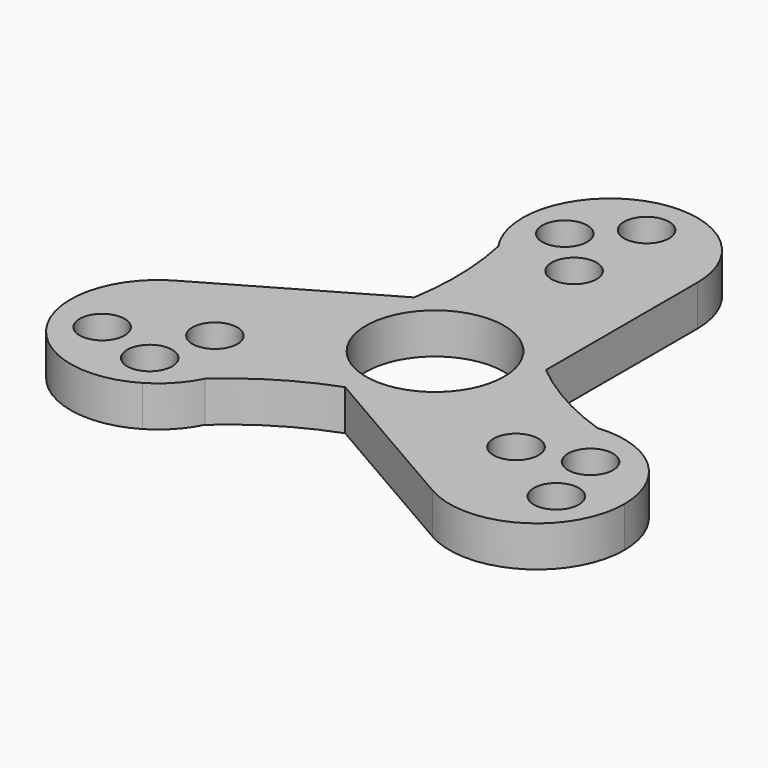
from build123d import *

# Parameters (mm, degrees)
F0_R     = 3.6
F0_R_2   = 11.05
F1_DEPTH = 6.5


# Not quite as in the source:
# - a feature names something its author has since deleted; it is built from what else it names


with BuildPart() as f1:
    # F0 (on Top) → F1 (new body)
    with BuildSketch(Plane.XY):
        with BuildLine():
            ThreePointArc((-23.0209464524, -29.3076083822), (-19.9383676627, -26.8167802289), (-17.6773098575, -23.5619170235))
            ThreePointArc((-17.6773098575, -23.5619170235), (-20.4709038775, -26.3215082368), (-23.0209464524, -29.3076083822))
        make_face()
        with BuildLine():
            ThreePointArc((-2.5600533635, -14.3957456382), (-1.63787321, -14.0667717582), (-0.7089513801, -13.7573460272))
            ThreePointArc((-0.7089513801, -13.7573460272), (-3.7381834506, -13.2395644299), (-6.5814605839, -12.0733226612))
            Line((-6.5814605839, -12.0733226612), (-2.5600533635, -14.3957456382))
        make_face()
        with BuildLine():
            ThreePointArc((-0.7089513801, -13.7573460272), (3.2568779095, -13.4262355322), (6.9693155956, -11.9926238203))
            ThreePointArc((6.9693155956, -11.9926238203), (3.0926272048, -12.7115843783), (-0.7089513801, -13.7573460272))
        make_face()
        with BuildLine():
            ThreePointArc((29.002813969, -3.3554863963), (22.1605329653, -5.9872334975), (17.5863384821, -11.7160769207))
            ThreePointArc((17.5863384821, -11.7160769207), (17.1389450218, -21.6742013703), (23.4307313902, -29.4058136055))
            ThreePointArc((23.4307313902, -29.4058136055), (37.4314802249, -29.4071108103), (44.4322291397, -17.282322802))
            ThreePointArc((44.4322291397, -17.282322802), (39.8127458528, -6.8897337985), (29.002813969, -3.3554863963))
        make_face()
        with Locations((24.2079713773, -13.6886037443)):
            Circle(F0_R, mode=Mode.SUBTRACT)
        with Locations((36.4874702709, -20.9787380615)):
            Circle(F0_R, mode=Mode.SUBTRACT)
        with Locations((33.9983616409, -11.0225966846)):
            Circle(F0_R, mode=Mode.SUBTRACT)
        with BuildLine():
            ThreePointArc((-23.0209464524, -29.3076083822), (-20.4709038775, -26.3215082368), (-17.6773098575, -23.5619170235))
            ThreePointArc((-17.6773098575, -23.5619170235), (-16.5669328393, -20.5090534106), (-16.1900430763, -17.2824658218))
            ThreePointArc((-16.1900430763, -17.2824658218), (-16.8601676515, -13.0029306649), (-18.8063889562, -9.1330843193))
            ThreePointArc((-18.8063889562, -9.1330843193), (-27.0153338433, -3.6471725985), (-36.8032431016, -4.9428716054))
            ThreePointArc((-36.8032431016, -4.9428716054), (-42.3755818337, -24.1754075155), (-23.0209464524, -29.3076083822))
        make_face()
        with Locations((-26.552398323, -23.5003339555)):
            Circle(F0_R, mode=Mode.SUBTRACT)
        with Locations((-36.419223994, -20.6778945734)):
            Circle(F0_R, mode=Mode.SUBTRACT)
        with Locations((-23.9660330315, -13.6886037443)):
            Circle(F0_R, mode=Mode.SUBTRACT)
        with BuildLine():
            ThreePointArc((-11.3063452022, 8.3060793433), (-9.4777201208, 10.4094594589), (-7.2686697166, 12.1089222888))
            Line((-7.2686697166, 12.1089222888), (-11.0034872924, 9.9526243561))
            ThreePointArc((-11.0034872924, 9.9526243561), (-11.1474831305, 9.1279846364), (-11.3063452022, 8.3060793433))
        make_face()
        with BuildLine():
            ThreePointArc((-13.8745275017, -0.137033899), (-12.3890775486, 4.023274448), (-11.3063452022, 8.3060793433))
            ThreePointArc((-11.3063452022, 8.3060793433), (-13.2731105164, 4.292175001), (-13.8745275017, -0.137033899))
        make_face()
        with BuildLine():
            ThreePointArc((6.7990177159, 12.5226532313), (9.6860598983, 9.0919172063), (12.891022892, 5.9561279205))
            ThreePointArc((12.891022892, 5.9561279205), (10.3843499056, 9.7397463301), (6.7990177159, 12.5226532313))
        make_face()
        with BuildLine():
            ThreePointArc((12.891022892, 5.9561279205), (13.810029624, 3.1522495359), (14.1209691729, 0.2180334624))
            Line((14.1209691729, 0.2180334624), (14.1209691729, 4.9018602452))
            ThreePointArc((14.1209691729, 4.9018602452), (13.5013908187, 5.4236214762), (12.891022892, 5.9561279205))
        make_face()
        with BuildLine():
            ThreePointArc((-11.4281301493, 27.3048605939), (-12.4782019744, 31.2955370079), (-13.8789707842, 35.1770310271))
            ThreePointArc((-13.8789707842, 35.1770310271), (-13.2461965273, 31.0564374771), (-11.4281301493, 27.3048605939))
        make_face()
        with BuildLine():
            ThreePointArc((6.7990177159, 12.5226532313), (10.3843499056, 9.7397463301), (12.891022892, 5.9561279205))
            ThreePointArc((12.891022892, 5.9561279205), (13.5013908187, 5.4236214762), (14.1209691729, 4.9018602452))
            Line((14.1209691729, 4.9018602452), (14.1209691729, 35.2180334624))
            ThreePointArc((14.1209691729, 35.2180334624), (4.2629861628, 21.8447879604), (-11.4281301493, 27.3048605939))
            ThreePointArc((-11.4281301493, 27.3048605939), (-10.3964763758, 18.6487931257), (-11.0034872924, 9.9526243561))
            Line((-11.0034872924, 9.9526243561), (-7.2686697166, 12.1089222888))
            ThreePointArc((-7.2686697166, 12.1089222888), (-0.2905931292, 14.2119827431), (6.7990177159, 12.5226532313))
        make_face()
        with BuildLine():
            ThreePointArc((6.9693155956, -11.9926238203), (12.2014668844, -6.8573870227), (14.1209691729, 0.2180334624))
            ThreePointArc((14.1209691729, 0.2180334624), (13.810029624, 3.1522495359), (12.891022892, 5.9561279205))
            ThreePointArc((12.891022892, 5.9561279205), (9.6860598983, 9.0919172063), (6.7990177159, 12.5226532313))
            ThreePointArc((6.7990177159, 12.5226532313), (-0.2905931292, 14.2119827431), (-7.2686697166, 12.1089222888))
            ThreePointArc((-7.2686697166, 12.1089222888), (-9.4777201208, 10.4094594589), (-11.3063452022, 8.3060793433))
            ThreePointArc((-11.3063452022, 8.3060793433), (-12.3890775486, 4.023274448), (-13.8745275017, -0.137033899))
            ThreePointArc((-13.8745275017, -0.137033899), (-11.8255695306, -7.0812961649), (-6.5814605839, -12.0733226612))
            ThreePointArc((-6.5814605839, -12.0733226612), (-3.7381834506, -13.2395644299), (-0.7089513801, -13.7573460272))
            ThreePointArc((-0.7089513801, -13.7573460272), (3.0926272048, -12.7115843783), (6.9693155956, -11.9926238203))
        make_face()
        with Locations((0.1209691729, 0.2180334624)):
            Circle(F0_R_2, mode=Mode.SUBTRACT)
        with BuildLine():
            ThreePointArc((-13.8745275017, -0.137033899), (-13.2731105164, 4.292175001), (-11.3063452022, 8.3060793433))
            ThreePointArc((-11.3063452022, 8.3060793433), (-11.1474831305, 9.1279846364), (-11.0034872924, 9.9526243561))
            Line((-11.0034872924, 9.9526243561), (-36.8032431016, -4.9428716054))
            ThreePointArc((-36.8032431016, -4.9428716054), (-27.0153338433, -3.6471725985), (-18.8063889562, -9.1330843193))
            ThreePointArc((-18.8063889562, -9.1330843193), (-16.0908458514, -4.7719029024), (-13.8745275017, -0.137033899))
        make_face()
        with BuildLine():
            Line((-2.5600533635, -14.3957456382), (-6.5814605839, -12.0733226612))
            ThreePointArc((-6.5814605839, -12.0733226612), (-11.8255695306, -7.0812961649), (-13.8745275017, -0.137033899))
            ThreePointArc((-13.8745275017, -0.137033899), (-16.0908458514, -4.7719029024), (-18.8063889562, -9.1330843193))
            ThreePointArc((-18.8063889562, -9.1330843193), (-16.8601676515, -13.0029306649), (-16.1900430763, -17.2824658218))
            ThreePointArc((-16.1900430763, -17.2824658218), (-16.5669328393, -20.5090534106), (-17.6773098575, -23.5619170235))
            ThreePointArc((-17.6773098575, -23.5619170235), (-10.5596558993, -18.2515569705), (-2.5600533635, -14.3957456382))
        make_face()
        with BuildLine():
            ThreePointArc((17.5863384821, -11.7160769207), (12.2698816763, -11.5493167715), (6.9693155956, -11.9926238203))
            ThreePointArc((6.9693155956, -11.9926238203), (3.2568779095, -13.4262355322), (-0.7089513801, -13.7573460272))
            ThreePointArc((-0.7089513801, -13.7573460272), (-1.63787321, -14.0667717582), (-2.5600533635, -14.3957456382))
            Line((-2.5600533635, -14.3957456382), (23.4307313902, -29.4058136055))
            ThreePointArc((23.4307313902, -29.4058136055), (17.1389450218, -21.6742013703), (17.5863384821, -11.7160769207))
        make_face()
        with BuildLine():
            Line((14.1209691729, 4.9018602452), (14.1209691729, 0.2180334624))
            ThreePointArc((14.1209691729, 0.2180334624), (12.2014668844, -6.8573870227), (6.9693155956, -11.9926238203))
            ThreePointArc((6.9693155956, -11.9926238203), (12.2698816763, -11.5493167715), (17.5863384821, -11.7160769207))
            ThreePointArc((17.5863384821, -11.7160769207), (22.1605329653, -5.9872334975), (29.002813969, -3.3554863963))
            ThreePointArc((29.002813969, -3.3554863963), (21.1797290943, 0.0844326658), (14.1209691729, 4.9018602452))
        make_face()
        with BuildLine():
            ThreePointArc((-11.4281301493, 27.3048605939), (4.2629861628, 21.8447879604), (14.1209691729, 35.2180334624))
            ThreePointArc((14.1209691729, 35.2180334624), (0.1004679333, 49.2180184516), (-13.8789707842, 35.1770310271))
            ThreePointArc((-13.8789707842, 35.1770310271), (-12.4782019744, 31.2955370079), (-11.4281301493, 27.3048605939))
        make_face()
        with Locations((0.1209691729, 28.0313078757)):
            Circle(F0_R, mode=Mode.SUBTRACT)
        with Locations((-7.0830557993, 35.1770310271)):
            Circle(F0_R, mode=Mode.SUBTRACT)
        with Locations((0.2946612417, 42.3107330219)):
            Circle(F0_R, mode=Mode.SUBTRACT)
    extrude(amount=F1_DEPTH)


solid = f1.part
